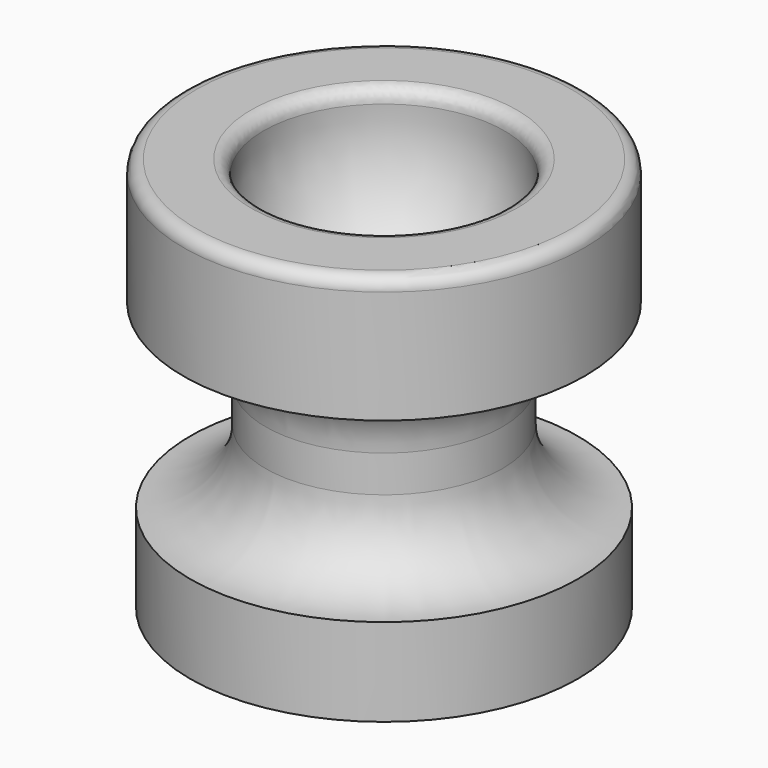
from build123d import *

# Parameters (mm, degrees)
F3_R = 5


# Not quite as in the source:
# - a feature of the source that left no trace in its solid (it failed there, or was rolled back) is left out


with BuildPart() as f2:
    # F0 (on Front) → F2 (revolve)
    with BuildSketch(Plane.XZ):
        with BuildLine():
            Line((38.9296258549, 0), (76.2161314487, 0))
            Line((76.2161314487, 0), (76.2161314487, 34.5504507422))
            ThreePointArc((76.2161314487, 34.5504507422), (55.3522757176, 42.613287739), (46.6280132532, 63.2093325257))
            Line((46.6280132532, 63.2093325257), (46.6280132532, 77.6744805479))
            ThreePointArc((46.6280132532, 77.6744805479), (56.3893375618, 99.0839330453), (78.9535716176, 105.7550236583))
            Line((78.9535716176, 105.7550236583), (78.9535716176, 155.2447585142))
            Line((78.9535716176, 155.2447585142), (46.4198933914, 155.2447585142))
            ThreePointArc((46.4198933914, 155.2447585142), (40.8771418071, 117.3123958387), (11.5445833653, 92.6306769252))
            Line((11.5445833653, 92.6306769252), (11.5445833653, 54.7694249827))
            ThreePointArc((11.5445833653, 54.7694249827), (32.356898751, 30.9446524602), (38.9296258549, 0))
        make_face()
    revolve(axis=Axis((0, 0, 66.4308094728), (0, 0, -1)))

    # F3
    f3_edges = [f2.edges().sort_by_distance(p)[0] for p in [
        (-78.953572, 0, 155.244759),
        (-46.419893, 0, 155.244759),
    ]]
    fillet(f3_edges, radius=F3_R)


solid = f2.part
